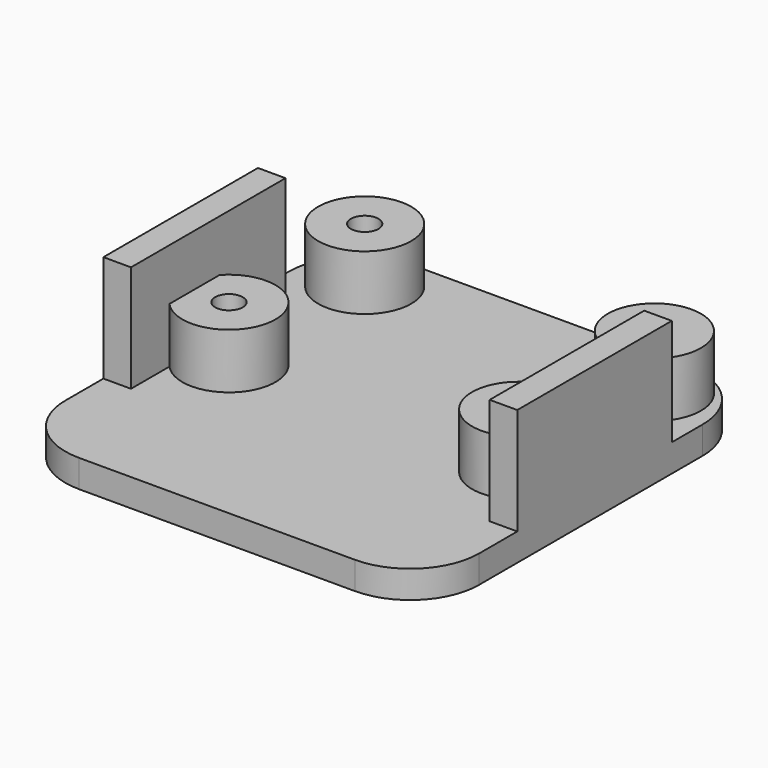
from build123d import *

# Parameters (mm, degrees)
F0_W     = 30
F0_H     = 30.25
F1_DEPTH = 2
F2_W     = 2
F2_H     = 14
F3_DEPTH = 7.75
F5_R     = 3.375
F6_DEPTH = 6
F4_R     = 1.875
F7_DEPTH = 4
F9_D     = 2
F9_DEPTH = 4
F9_START = 4
F9_TIP   = 0.600860619
F10_R    = 5


with BuildPart() as f1:
    # F0 (on Top) → F1 (new body)
    with BuildSketch(Plane.XY):
        Rectangle(F0_W, F0_H)
    extrude(amount=F1_DEPTH)

    # F2 (on face) → F3 (join)
    with BuildSketch(Plane.XY.offset(2)):
        with Locations((-14, 0.325)):
            Rectangle(F2_W, F2_H)
        with Locations((14, 0.325)):
            Rectangle(F2_W, F2_H)
    extrude(amount=F3_DEPTH)

    # F5 (on face) → F6 (join)
    with BuildSketch(Plane(origin=(0, 0, 0), x_dir=(1, 0, 0), z_dir=(0, 0, -1))):
        with Locations((10.5, -11.375)):
            Circle(F5_R)
        with Locations((-10.5, -11.375)):
            Circle(F5_R)
        with Locations((-10.5, 0.925)):
            Circle(F5_R)
        with Locations((10.5, 0.925)):
            Circle(F5_R)
    extrude(amount=-F6_DEPTH)

    # F4 (on face) → F7 (cut)
    with BuildSketch(Plane(origin=(0, 0, 0), x_dir=(1, 0, 0), z_dir=(0, 0, -1))):
        with Locations((-10.5, -11.375)):
            Circle(F4_R)
        with Locations((-10.5, 0.925)):
            Circle(F4_R)
        with Locations((10.5, -11.375)):
            Circle(F4_R)
        with Locations((10.5, 0.925)):
            Circle(F4_R)
    extrude(amount=-F7_DEPTH, mode=Mode.SUBTRACT)

    # F9
    # its depths count from where the whole tool has entered the part; down to there all is cleared
    with Locations(Plane(origin=(0, 0, 0), x_dir=(1, 0, 0), z_dir=(0, 0, -1)).offset(-F9_START)):
        with Locations((-10.5, 0.925), (-10.5, -11.375), (10.5, -11.375), (10.5, 0.925)):
            Hole(F9_D / 2, depth=F9_DEPTH)
            with Locations((0, 0, -(F9_DEPTH + F9_TIP / 2))):  # 118° drill point
                Cone(0, F9_D / 2, F9_TIP, mode=Mode.SUBTRACT)

    # F10
    f10_edges = [f1.edges().sort_by_distance(p)[0] for p in [
        (-15, -15.125, 1),
        (15, -15.125, 1),
        (15, 15.125, 1),
        (-15, 15.125, 1),
    ]]
    fillet(f10_edges, radius=F10_R)


solid = f1.part
